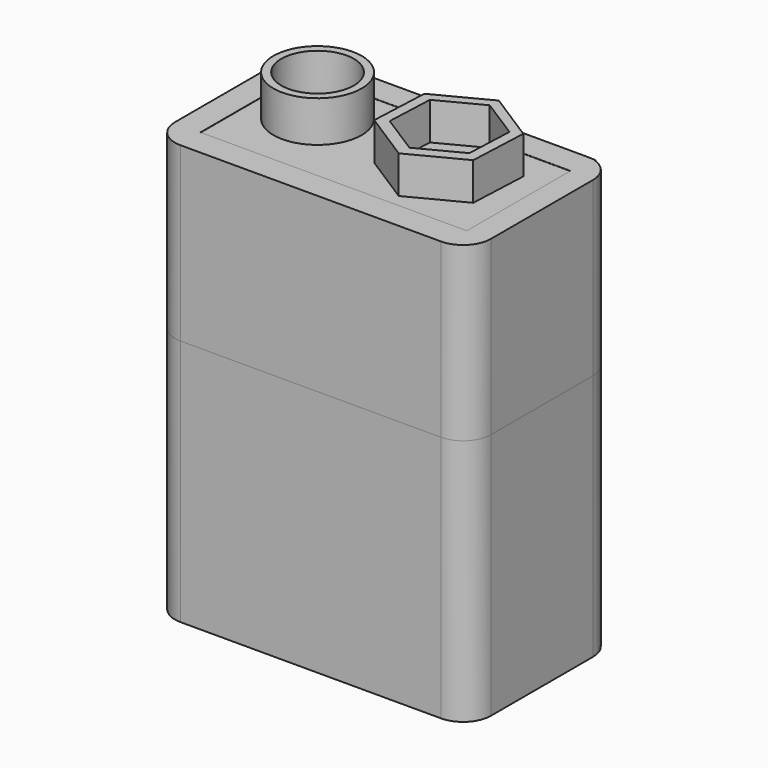
from build123d import *

# Parameters (mm, degrees)
F0_W      = 55.313270539
F0_H      = 75.847633183
F1_DEPTH  = 31.75
F2_R      = 5.08
F3_R      = 8.0658325131
F3_R_2    = 6.6237237861
F4_DEPTH  = 8.636
F5_R      = 10.2149655363
F6_DEPTH  = 31.75
F9_DEPTH  = 38.608
F11_DEPTH = 38.862
F13_DEPTH = 27.94
F14_W     = 57.7289052308
F14_H     = 33.4668345749
F15_DEPTH = 31.496
F16_DEPTH = 45.212
F17_R     = 5.08
F17_2_R   = 5.08
F18_W     = 48.6534815282
F18_H     = 23.6792610958
F19_DEPTH = 31.75
F20_W     = 49.7737694532
F20_H     = 77.0872496068
F21_DEPTH = 29.21


# Not quite as in the source:
# - a fillet or chamfer that OpenCascade refuses, or shapes differently, is made with other operations: its cross-section is extruded or revolved along the edge and cut away or added


with BuildPart() as f1:
    # F0 (on Front) → F1 (new body)
    with BuildSketch(Plane.XZ):
        with Locations((0.8324738592, -7.3072724044)):
            Rectangle(F0_W, F0_H)
    extrude(amount=F1_DEPTH)

    # F2
    f2_edges = [f1.edges().sort_by_distance(p)[0] for p in [
        (28.489109, -31.75, -7.307272),
        (-26.824161, -31.75, -7.307272),
        (28.489109, 0, -7.307272),
        (-26.824161, 0, -7.307272),
    ]]
    fillet(f2_edges, radius=F2_R)



with BuildPart() as f4:
    # F3 (on face) → F4 (new body)
    with BuildSketch(Plane.XY.offset(30.6165441871)):
        with Locations((-12.2096184641, -15.2620235458)):
            Circle(F3_R)
        with Locations((-12.2096184641, -15.2620235458)):
            Circle(F3_R_2, mode=Mode.SUBTRACT)
    extrude(amount=F4_DEPTH)


with BuildPart() as f1_1:
    add(f1.part)

    add(f4.part)  # F6 merges F4
    # F5 (on Top) → F6 (join)
    with BuildSketch(Plane.XY):
        with Locations((-12.0246242732, -15.0770293549)):
            Circle(F5_R)
    extrude(amount=F6_DEPTH)

    # F7: fillet of radius 3.0660512242 on 1 edges, made by hand

    # F7_s1 → F7_t2 (revolve)
    with BuildSketch(Plane.XZ.offset(15.0770293549)):
        with BuildLine():
            ThreePointArc((-1.8096587369, 31.75), (-0.7475631061, 30.9143733613), (0.5706238273, 30.6165441871))
            Line((0.5706238273, 30.6165441871), (-1.8096587369, 30.6165441871))
            Line((-1.8096587369, 30.6165441871), (-1.8096587369, 31.75))
        make_face()
    revolve(axis=Axis((-12.0246242732, -15.0770293549, 30.6165441871), (0, 0, -1)))

    # F8 (on Top) → F9 (join)
    with BuildSketch(Plane.XY):
        Polygon((21.3451305674, -21.6504897434), (21.8293182552, -10.8221620321), (12.6938052206, -4.9886793386), (3.0741044982, -9.9835243564), (2.5899168104, -20.8118520677), (11.725429845, -26.6453347612), align=None)
    extrude(amount=F9_DEPTH)

    # F10 (on Top) → F11 (cut)
    with BuildSketch(Plane.XY):
        Polygon((19.9244704443, -11.6050673129), (12.5796077773, -6.9372830912), (4.8647567285, -10.9642286373), (4.4947683466, -19.6589584051), (11.8396310136, -24.3267426267), (19.5544820624, -20.2997970807), align=None)
    extrude(amount=F11_DEPTH, mode=Mode.SUBTRACT)

    # F12 (on Top) → F13 (join)
    with BuildSketch(Plane.XY):
        Polygon((19.2986911239, -20.0054645374), (19.7943821549, -11.7471329868), (12.8903027548, -7.1886861861), (5.4905323236, -10.8885709361), (4.9948412925, -19.1469024867), (11.8989206926, -23.7053492873), align=None)
    extrude(amount=F13_DEPTH)


with BuildPart() as f15:
    # F14 (on Top) → F15 (new body)
    with BuildSketch(Plane.XY):
        with Locations((1.1070892215, -16.7334172875)):
            Rectangle(F14_W, F14_H)
    extrude(amount=F15_DEPTH)

    # F17
    f17_edges = [f15.edges().sort_by_distance(p)[0] for p in [
        (29.971542, -33.466835, 15.748),
        (-27.757363, -33.466835, 15.748),
        (-27.757363, 0, 15.748),
        (29.971542, 0, 15.748),
    ]]
    fillet(f17_edges, radius=F17_R)


with BuildPart() as f16:
    # F14 (on Top) → F16 (new body)
    with BuildSketch(Plane.XY):
        with Locations((1.1070892215, -16.7334172875)):
            Rectangle(F14_W, F14_H)
    extrude(amount=-F16_DEPTH)

    # F17#2
    f17_2_edges = [f16.edges().sort_by_distance(p)[0] for p in [
        (29.971542, -33.466835, -22.606),
        (-27.757363, -33.466835, -22.606),
        (-27.757363, 0, -22.606),
        (29.971542, 0, -22.606),
    ]]
    fillet(f17_2_edges, radius=F17_2_R)


with BuildPart() as f19_tool:
    # F18 (on Top) → F19 (new body)
    with BuildSketch(Plane.XY):
        with Locations((1.3874573633, -16.7419775389)):
            Rectangle(F18_W, F18_H)
    extrude(amount=F19_DEPTH)


with BuildPart() as f1_2:
    add(f1_1.part)

    # F19: cut by f19_tool
    add(f19_tool.part, mode=Mode.SUBTRACT)


with BuildPart() as f15_1:
    add(f15.part)

    # F19: cut by f19_tool
    add(f19_tool.part, mode=Mode.SUBTRACT)


with BuildPart() as f21:
    # F20 (on Front) → F21 (new body)
    with BuildSketch(Plane.XZ):
        with Locations((1.4411928132, -7.0859994739)):
            Rectangle(F20_W, F20_H)
    extrude(amount=F21_DEPTH)


solid = Compound([f16.part, f1_2.part, f15_1.part, f21.part])
